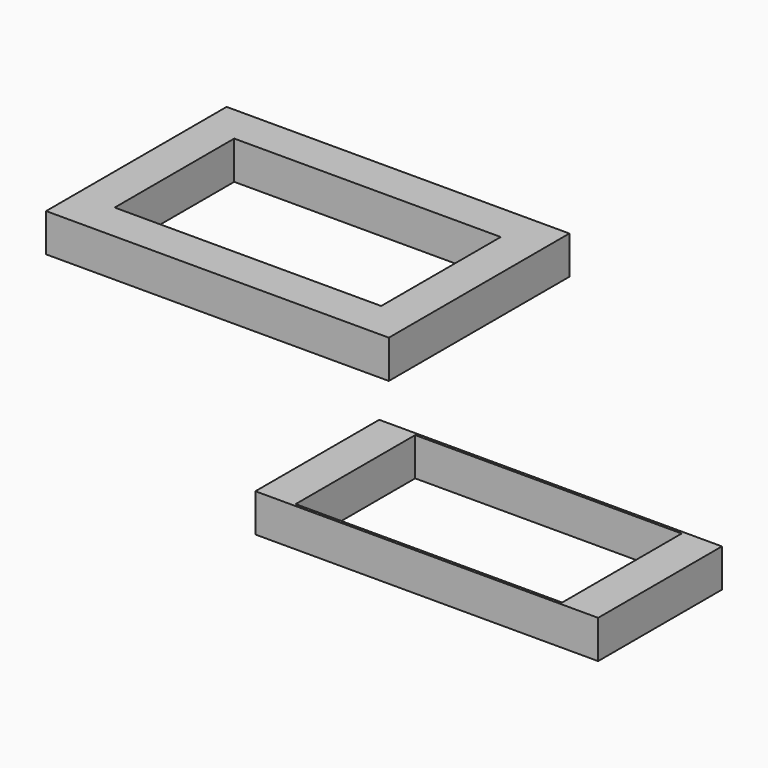
from build123d import *

# Parameters (mm, degrees)
F0_W     = 28.5496
F0_H     = 12.8888987312
F0_W_2   = 22.1996
F0_H_2   = 12.446
F1_DEPTH = 3.175
F0_H_3   = 18.796
F2_DEPTH = 3.175


with BuildPart() as f1:
    # F0 (on Top) → F1 (new body)
    with BuildSketch(Plane.XY):
        Rectangle(F0_W, F0_H)
        Rectangle(F0_W_2, F0_H_2, mode=Mode.SUBTRACT)
    extrude(amount=F1_DEPTH)


with BuildPart() as f2:
    # F0 (on Top) → F2 (new body)
    with BuildSketch(Plane.XY):
        with Locations((-35.2845547821, 25.2655620637)):
            Rectangle(F0_W, F0_H_3)
        with Locations((-35.2845547821, 25.2655620637)):
            Rectangle(F0_W_2, F0_H_2, mode=Mode.SUBTRACT)
    extrude(amount=F2_DEPTH)


solid = Compound([f1.part, f2.part])
